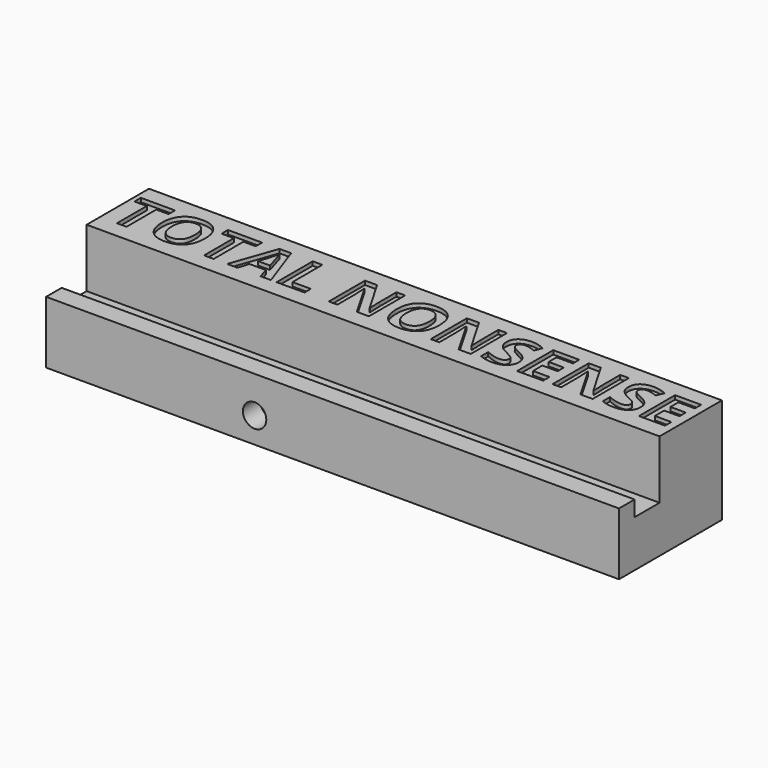
from build123d import *

# Parameters (mm, degrees)
F1_DEPTH     = 147
F3_DEPTH     = 12.001
F4_TEXT_SIZE = 16.25
F5_DEPTH     = 1
F7_DEPTH     = 9.9
F8_R         = 3
F9_DEPTH     = 5.6


# Not quite as in the source:
# - Text() gives the source's letters only with a copy of the font that has no kerning and outlines rounded to 1/6400 em; it was checked with that copy


with BuildPart() as f1:
    # F0 (on Right) → F1 (new body)
    with BuildSketch(Plane.YZ):
        Polygon((-33, 16), (-33, 0), (0, 0), (0, 27), (-20, 27), (-20, 12), (-28, 12), (-28, 16), align=None)
    extrude(amount=F1_DEPTH)

    # F2 (on face) → F3 (cut, through all)
    with BuildSketch(Plane.XY.offset(12)):
        with BuildLine():
            Line((65.55, -26.05), (82.85, -26.05))
            ThreePointArc((82.85, -26.05), (84.9, -24), (82.85, -21.95))
            Line((82.85, -21.95), (65.55, -21.95))
            ThreePointArc((65.55, -21.95), (63.5, -24), (65.55, -26.05))
        make_face()
    extrude(amount=-F3_DEPTH, mode=Mode.SUBTRACT)

    # F4 (on face) → F5 (cut)
    with BuildSketch(Plane.XY.offset(27)):
        with Locations((0.8697265625, -15.7)):
            Text('TOTAL NONSENSE', F4_TEXT_SIZE, font='Open Sans', font_style=FontStyle.BOLD, text_align=(TextAlign.LEFT, TextAlign.BOTTOM))
    extrude(amount=-F5_DEPTH, mode=Mode.SUBTRACT)

    # F6 (on face) → F7 (cut)
    with BuildSketch(Plane(origin=(0, 0, 0), x_dir=(1, 0, 0), z_dir=(0, 0, -1))):
        with BuildLine():
            Line((86.9, 27.4), (41.5, 27.4))
            ThreePointArc((41.5, 27.4), (39.3786796564, 26.5213203436), (38.5, 24.4))
            Line((38.5, 24.4), (38.5, 23.6))
            ThreePointArc((38.5, 23.6), (39.3786796564, 21.4786796564), (41.5, 20.6))
            Line((41.5, 20.6), (44.9367240071, 20.6))
            Line((44.9367240071, 20.6), (44.9367240071, 0))
            Line((44.9367240071, 0), (51.2367240071, 0))
            Line((51.2367240071, 0), (51.2367240071, 20.6))
            Line((51.2367240071, 20.6), (86.9, 20.6))
            ThreePointArc((86.9, 20.6), (89.0213203436, 21.4786796564), (89.9, 23.6))
            Line((89.9, 23.6), (89.9, 24.4))
            ThreePointArc((89.9, 24.4), (89.0213203436, 26.5213203436), (86.9, 27.4))
        make_face()
    extrude(amount=-F7_DEPTH, mode=Mode.SUBTRACT)

    # F8 (on face) → F9 (cut, through all)
    with BuildSketch(Plane.XZ.offset(33)):
        with Locations((53.5, 6.6)):
            Circle(F8_R)
    extrude(amount=-F9_DEPTH, mode=Mode.SUBTRACT)


solid = f1.part
